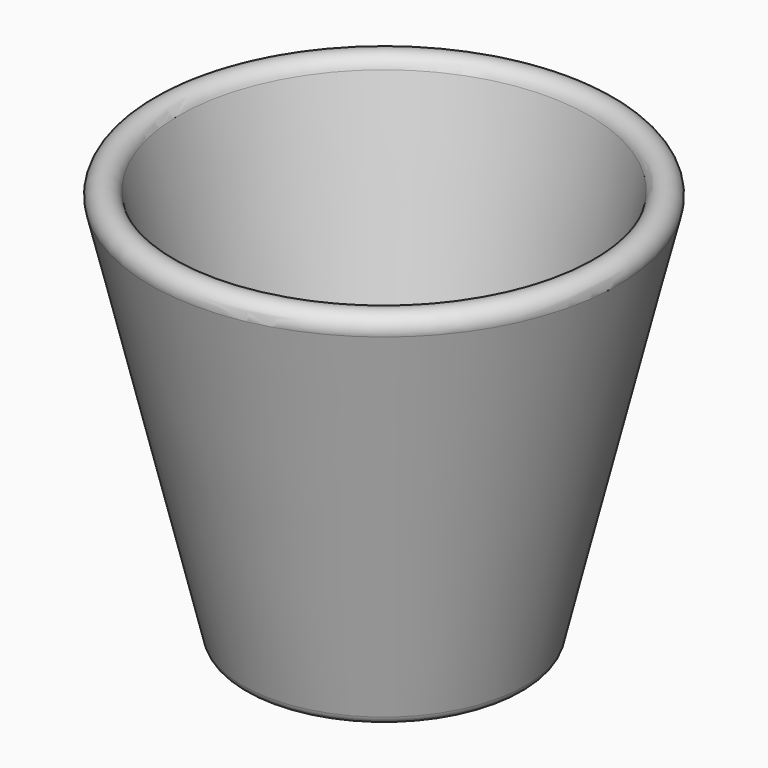
from build123d import *

# Parameters (mm, degrees)
F2_TEXT_SIZE = 13.6915180418
F4_R         = 27.5355943056
F5_DEPTH     = 0.5


# Not quite as in the source:
# - Text() gives the source's letters only with a copy of the font that has no kerning and outlines rounded to 1/6400 em; it was checked with that copy


with BuildPart() as f1:
    # F0 (on Right) → F1 (revolve)
    with BuildSketch(Plane.YZ):
        with BuildLine():
            Line((-34.9993163568, 0), (-27.5355943056, 0))
            ThreePointArc((-27.5355943056, 0), (-14.3796640587, 6.1798938421), (0, 8.3))
            Line((0, 8.3), (0, 16.3))
            Line((0, 16.3), (-23.6294222003, 16.3))
            ThreePointArc((-23.6294222003, 16.3), (-31.0503636399, 18.8697493061), (-35.2929785603, 25.4783953084))
            Line((-35.2929785603, 25.4783953084), (-55, 106.9405348972))
            ThreePointArc((-55, 106.9405348972), (-59.8283870172, 109.88785212), (-62.77570424, 105.0594651028))
            Line((-62.77570424, 105.0594651028), (-37.9152054468, 2.2945988271))
            ThreePointArc((-37.9152054468, 2.2945988271), (-36.8545517167, 0.6424373265), (-34.9993163568, 0))
        make_face()
    revolve(axis=Axis((0, 0, 8.15), (0, 0, -1)))

    # F2 (on face) → F3 (join, up to the next surface of F1)
    with BuildSketch(Plane(origin=(0, 0, 0), x_dir=(1, 0, 0), z_dir=(0, 0, -1))):
        with Locations((-25.74005723, -3.6771511659)):
            Text("K&D '17", F2_TEXT_SIZE, font='Open Sans', font_style=FontStyle.BOLD, text_align=(TextAlign.LEFT, TextAlign.BOTTOM))
    extrude(until=Until.NEXT, dir=(0, 0, 1))

    # F4 (on face) → F5 (cut)
    with BuildSketch(Plane(origin=(0, 0, 0), x_dir=(1, 0, 0), z_dir=(0, 0, -1))):
        Circle(F4_R)
    extrude(amount=-F5_DEPTH, mode=Mode.SUBTRACT)


solid = f1.part
